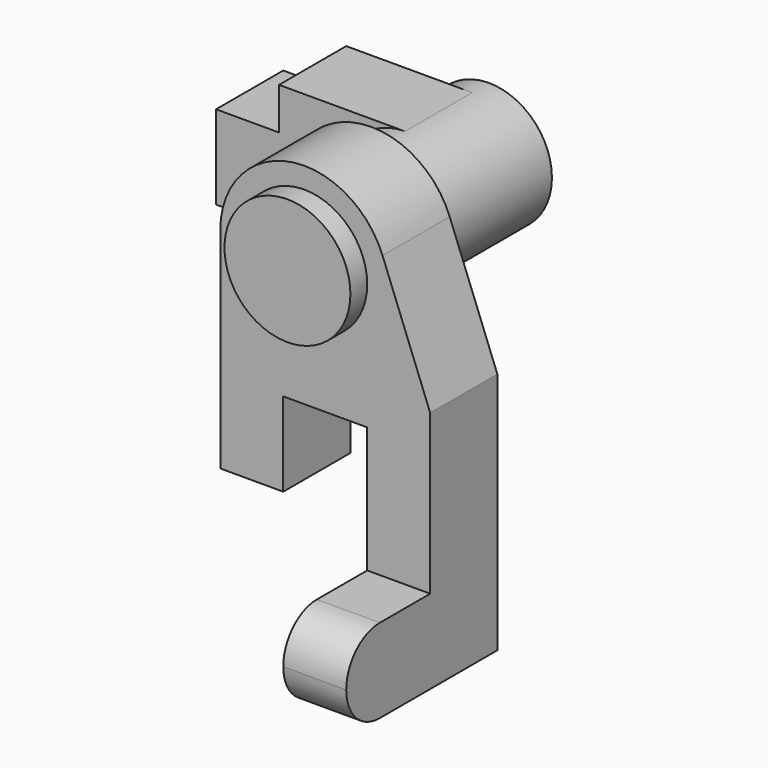
from build123d import *

# Parameters (mm, degrees)
F1_DEPTH      = 20
F2_R          = 15
F3_DEPTH      = 5
F3_DEPTH_BACK = 55
F4_W          = 15
F4_H          = 20
F5_DEPTH      = 25
F6_R          = 9.99999
F7_W          = 15
F7_H          = 10
F8_DEPTH      = 25
F9_DEPTH      = 25
F10_DEPTH     = 5


# Not quite as in the source:
# - a fillet or chamfer is up to 0.001 mm smaller than in the source, because OpenCascade refuses the exact size


with BuildPart() as f1:
    # F0 (on Front) → F1 (new body)
    with BuildSketch(Plane.XZ):
        with BuildLine():
            ThreePointArc((18.649535318, 7.2245991185), (19.659485069, 3.6748669119), (20, 0))
            ThreePointArc((20, 0), (0, -20), (-20, 0))
            Line((-20, 0), (-20, -50))
            Line((-20, -50), (-5, -50))
            Line((-5, -50), (-5, -30))
            Line((-5, -30), (15, -30))
            Line((15, -30), (15, -80))
            Line((15, -80), (30, -80))
            Line((30, -80), (30, -22.0754199539))
            Line((30, -22.0754199539), (18.649535318, 7.2245991185))
        make_face()
        with BuildLine():
            ThreePointArc((-20, 0), (0, -20), (20, 0))
            ThreePointArc((20, 0), (19.659485069, 3.6748669119), (18.649535318, 7.2245991185))
            ThreePointArc((18.649535318, 7.2245991185), (-3.6748669119, 19.659485069), (-20, 0))
        make_face()
    extrude(amount=-F1_DEPTH)

    # F2 (on face) → F3 (join, two sides)
    with BuildSketch(Plane.XZ) as f3_sk:
        Circle(F2_R)
    extrude(amount=F3_DEPTH)
    extrude(f3_sk.sketch, amount=-F3_DEPTH_BACK)

    # F4 (on face) → F5 (join)
    with BuildSketch(Plane.XZ):
        with Locations((22.5, -70)):
            Rectangle(F4_W, F4_H)
    extrude(amount=F5_DEPTH)

    # F6 (radius 10 in the source; OpenCascade refuses exactly that, so slightly less here)
    f6_edges = [f1.edges().sort_by_distance(p)[0] for p in [
        (22.5, -25, -60),
        (22.5, -25, -80),
    ]]
    fillet(f6_edges, radius=F6_R)

    # F7 (on face) → F8 (join)
    with BuildSketch(Plane(origin=(0, 55, 0), x_dir=(-1, 0, 0), z_dir=(0, 1, 0))):
        with Locations((37.5, 10)):
            Rectangle(F7_W, F7_H)
        with BuildLine():
            Line((30, 15), (0, 15))
            ThreePointArc((0, 15), (10.6066017178, 10.6066017178), (15, 0))
            ThreePointArc((15, 0), (10.6066017178, -10.6066017178), (0, -15))
            Line((0, -15), (45, -15))
            Line((45, -15), (45, 5))
            Line((45, 5), (30, 5))
            Line((30, 5), (30, 15))
        make_face()
    extrude(amount=-F8_DEPTH)

    # F7 (on face) → F9 (cut)
    with BuildSketch(Plane(origin=(0, 55, 0), x_dir=(-1, 0, 0), z_dir=(0, 1, 0))):
        with Locations((37.5, 10)):
            Rectangle(F7_W, F7_H)
    extrude(amount=-F9_DEPTH, mode=Mode.SUBTRACT)

    # F7 (on face) → F10 (cut)
    with BuildSketch(Plane(origin=(0, 55, 0), x_dir=(-1, 0, 0), z_dir=(0, 1, 0))):
        with Locations((37.5, 10)):
            Rectangle(F7_W, F7_H)
        with BuildLine():
            Line((30, 15), (0, 15))
            ThreePointArc((0, 15), (10.6066017178, 10.6066017178), (15, 0))
            ThreePointArc((15, 0), (10.6066017178, -10.6066017178), (0, -15))
            Line((0, -15), (45, -15))
            Line((45, -15), (45, 5))
            Line((45, 5), (30, 5))
            Line((30, 5), (30, 15))
        make_face()
    extrude(amount=-F10_DEPTH, mode=Mode.SUBTRACT)


solid = f1.part
